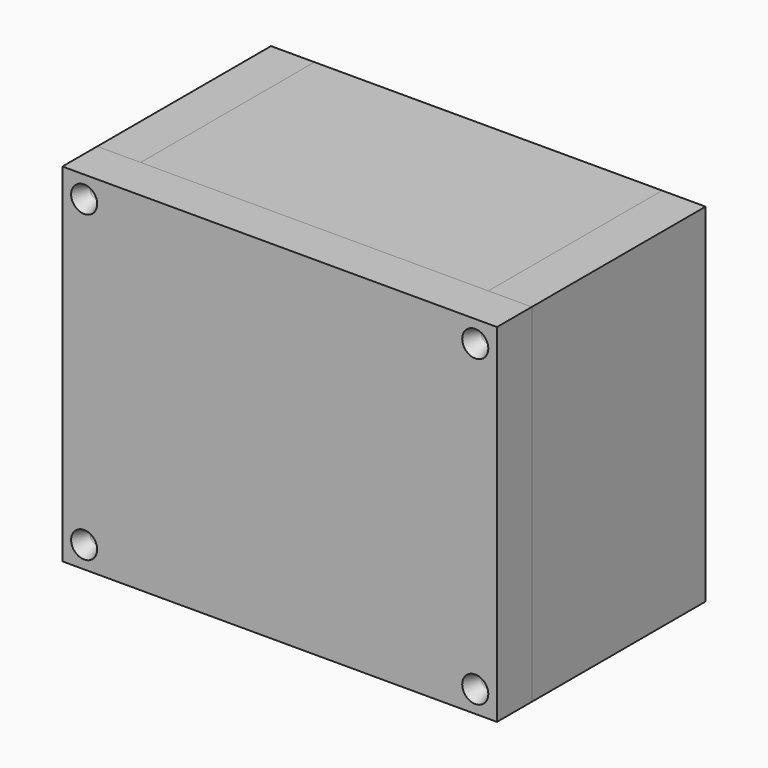
from build123d import *

# Parameters (mm, degrees)
F0_W             = 80
F0_H             = 10
F4_DEPTH         = 50
F2_W             = 80
F2_H             = 10
F5_W             = 10
F5_H             = 80
F6_DEPTH         = 100
F8_D             = 3
F8_CSINK_D       = 6
F8_CSINK_ANGLE   = 45
F8_2_D           = 3
F8_2_CSINK_D     = 6
F8_2_CSINK_ANGLE = 45


with BuildPart() as f4:
    # F0 (on Front) → F4 (new body)
    with BuildSketch(Plane.XZ):
        Polygon((-19.2272488975, 34.9881720543), (-19.2272488975, 44.9881720543), (-29.2272488975, 44.9881720543), (-29.2272488975, -35.0118279457), (-19.2272488975, -35.0118279457), (-19.2272488975, -25.0118279457), align=None)
        Polygon((70.7727511025, 44.9881720543), (60.7727511025, 44.9881720543), (60.7727511025, 34.9881720543), (60.7727511025, -25.0118279457), (60.7727511025, -35.0118279457), (70.7727511025, -35.0118279457), align=None)
        with Locations((20.7727511025, -30.0118279457)):
            Rectangle(F0_W, F0_H)
    extrude(amount=F4_DEPTH)

    # F8 (through all)
    with Locations(Plane.XZ.offset(60)):
        with Locations((-24.2272488975, 39.9881720543), (65.7727511025, 39.9881720543), (65.7727511025, -30.0118279457), (-24.2272488975, -30.0118279457)):
            CounterSinkHole(F8_D / 2, F8_CSINK_D / 2, counter_sink_angle=F8_CSINK_ANGLE)


with BuildPart() as f4b:
    # F2 (on face) → F4, piece 2 (new body)
    with BuildSketch(Plane.XZ):
        with Locations((20.7727511025, 39.9881720543)):
            Rectangle(F2_W, F2_H)
    extrude(amount=F4_DEPTH)


with BuildPart() as f6:
    # F5 (on face) → F6 (new body)
    with BuildSketch(Plane(origin=(-29.2272488975, 0, 0), x_dir=(0, -1, 0), z_dir=(-1, 0, 0))):
        with Locations((55, 4.9881720543)):
            Rectangle(F5_W, F5_H)
    extrude(amount=-F6_DEPTH)

    # F8#2 (through all)
    with Locations(Plane.XZ.offset(60)):
        with Locations((-24.2272488975, 39.9881720543), (65.7727511025, 39.9881720543), (65.7727511025, -30.0118279457), (-24.2272488975, -30.0118279457)):
            CounterSinkHole(F8_2_D / 2, F8_2_CSINK_D / 2, counter_sink_angle=F8_2_CSINK_ANGLE)


solid = Compound([f4.part, f4b.part, f6.part])
